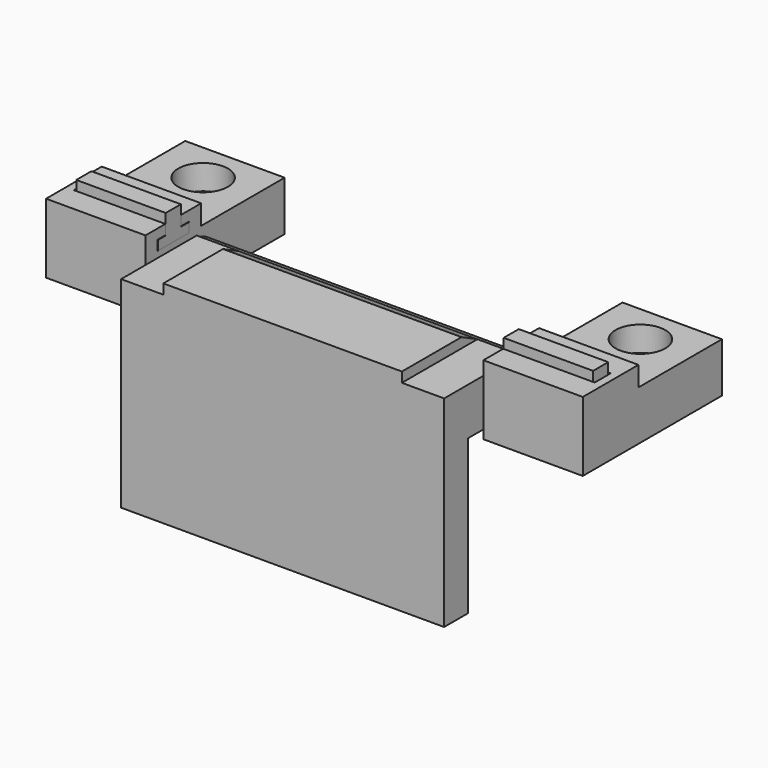
from build123d import *

# Parameters (mm, degrees)
F0_W           = 20
F0_H           = 35
F1_DEPTH       = 10
F3_D           = 5.5
F3_CBORE_D     = 10
F3_CBORE_DEPTH = 5
F5_DEPTH       = 20
F6_DEPTH       = 18
F8_DEPTH       = 1.6
F4_R           = 1.5
F9_DEPTH       = 4
F11_R          = 1.5
F12_DEPTH      = 38
F12_DEPTH_BACK = 38
F14_DEPTH      = 32.5
F16_W          = 65
F16_H          = 19
F17_DEPTH      = 0.5
F18_W          = 48
F18_H          = 19
F19_DEPTH      = 2
F20_SIZE2      = 2
F20_SIZE       = 4


# Not quite as in the source:
# - a feature names something its author has since deleted; it is built from what else it names


with BuildPart() as f1:
    # F0 (on Top) → F1 (new body)
    with BuildSketch(Plane.XY):
        with Locations((-44, 17.5)):
            Rectangle(F0_W, F0_H)
    extrude(amount=F1_DEPTH)

    # F3 (through all)
    with Locations(Plane.XY.offset(10)):
        with Locations((-44, 27)):
            CounterBoreHole(F3_D / 2, F3_CBORE_D / 2, F3_CBORE_DEPTH)

    # F4 (on face) → F5 (join, through all)
    with BuildSketch(Plane.YZ.offset(-34)):
        Polygon((0, 14), (0, 10), (3, 10), (3, 12), (5, 12), (5, 14), align=None)
        Polygon((11, 10), (14, 10), (14, 14), (9, 14), (9, 12), (11, 12), align=None)
    extrude(amount=-F5_DEPTH)

    # F7 (on face) → F8 (join)
    with BuildSketch(Plane(origin=(-54, 0, 0), x_dir=(0, -1, 0), z_dir=(-1, 0, 0))):
        Polygon((-5, 14), (-9, 14), (-9, 12), (-11, 12), (-11, 10), (-3, 10), (-3, 12), (-5, 12), align=None)
    extrude(amount=-F8_DEPTH)

    # F4 (on face) → F9 (cut)
    with BuildSketch(Plane.YZ.offset(-34)):
        with Locations((11, 5)):
            Circle(F4_R)
    extrude(amount=-F9_DEPTH, mode=Mode.SUBTRACT)


with BuildPart() as f6:
    # F4 (on face) → F6 (new body)
    with BuildSketch(Plane.YZ.offset(-34)):
        Polygon((3.1, 11.9), (3.1, 10), (7, 10), (10.9, 10), (10.9, 11.9), (8.9, 11.9), (8.9, 15.9), (7, 15.9), (5.1, 15.9), (5.1, 11.9), align=None)
    extrude(amount=-F6_DEPTH)


with BuildPart() as f10_1:
    # F10: instance of F1
    add(f1.part.mirror(Plane.YZ))


with BuildPart() as f10_2:
    # F10: instance of F6
    add(f6.part.mirror(Plane.YZ))


with BuildPart() as f12:
    # F11 (on Right) → F12 (new body, two sides)
    with BuildSketch(Plane.YZ) as f12_sk:
        with Locations((11, 5)):
            Circle(F11_R)
    extrude(amount=F12_DEPTH)
    extrude(f12_sk.sketch, amount=-F12_DEPTH_BACK)


with BuildPart() as f14:
    # F13 (on Right) → F14 (new body, symmetric)
    with BuildSketch(Plane.YZ):
        with BuildLine():
            Line((0, 0.5), (11, 0.5))
            ThreePointArc((11, 0.5), (6.5, 5), (11, 9.5))
            Line((11, 9.5), (-8, 9.5))
            Line((-8, 9.5), (-8, -30.5))
            Line((-8, -30.5), (-2, -30.5))
            Line((-2, -30.5), (-2, 0.5))
            Line((-2, 0.5), (0, 0.5))
        make_face()
        with BuildLine():
            ThreePointArc((11, 9.5), (6.5, 5), (11, 0.5))
            ThreePointArc((11, 0.5), (14.1819805153, 1.8180194847), (15.5, 5))
            ThreePointArc((15.5, 5), (14.1819805153, 8.1819805153), (11, 9.5))
        make_face()
    extrude(amount=F14_DEPTH, both=True)

    # F15: cut F12
    add(f12.part, mode=Mode.SUBTRACT)

    # F16 (on face) → F17 (join, through all)
    with BuildSketch(Plane.XY.offset(9.5)):
        with Locations((0, 1.5)):
            Rectangle(F16_W, F16_H)
    extrude(amount=F17_DEPTH)

    # F18 (on face) → F19 (join)
    with BuildSketch(Plane.XY.offset(10)):
        with Locations((0, 1.5)):
            Rectangle(F18_W, F18_H)
    extrude(amount=F19_DEPTH)

    # F20
    f20_edges = [f14.edges().sort_by_distance(p)[0] for p in [
        (0, 11, 12),
    ]]
    f20_side = f14.faces().sort_by_distance((0, 1.5, 12))[0]
    chamfer(f20_edges, length=F20_SIZE, length2=F20_SIZE2, reference=f20_side)


solid = Compound([f1.part, f6.part, f10_1.part, f10_2.part, f12.part, f14.part])
